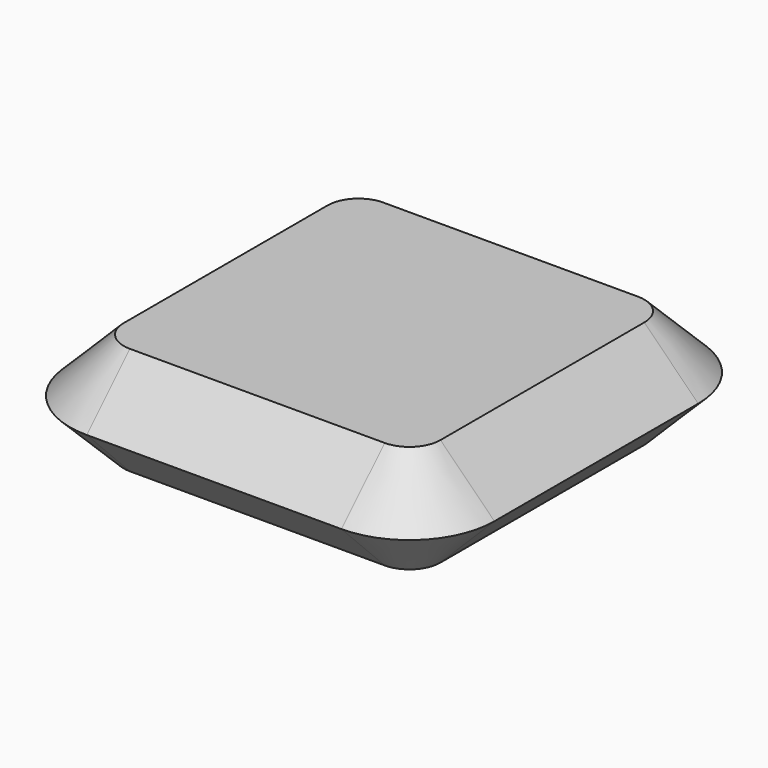
from build123d import *

# Parameters (mm, degrees)
F1_DEPTH = 25.4
F2_SIZE  = 12.7
F3_SIZE  = 12.69999


# Not quite as in the source:
# - a fillet or chamfer is up to 0.001 mm smaller than in the source, because OpenCascade refuses the exact size


with BuildPart() as f1:
    # F0 (on Top) → F1 (new body)
    with BuildSketch(Plane.XY):
        with BuildLine():
            Line((-30, -50), (30, -50))
            ThreePointArc((30, -50), (44.1421356237, -44.1421356237), (50, -30))
            Line((50, -30), (50, 30))
            ThreePointArc((50, 30), (44.1421356237, 44.1421356237), (30, 50))
            Line((30, 50), (-30, 50))
            ThreePointArc((-30, 50), (-44.1421356237, 44.1421356237), (-50, 30))
            Line((-50, 30), (-50, -30))
            ThreePointArc((-50, -30), (-44.1421356237, -44.1421356237), (-30, -50))
        make_face()
    extrude(amount=F1_DEPTH)

    # F2
    f2_edges = [f1.edges().sort_by_distance(p)[0] for p in [
        (0, -50, 25.4),
        (44.142136, -44.142136, 25.4),
        (50, 0, 25.4),
        (44.142136, 44.142136, 25.4),
        (0, 50, 25.4),
        (-44.142136, 44.142136, 25.4),
        (-50, 0, 25.4),
        (-44.142136, -44.142136, 25.4),
    ]]
    chamfer(f2_edges, length=F2_SIZE)

    # F3 (size 12.7 in the source; OpenCascade refuses exactly that, so slightly less here)
    f3_edges = [f1.edges().sort_by_distance(p)[0] for p in [
        (0, -50, 0),
        (44.142136, -44.142136, 0),
        (50, 0, 0),
        (44.142136, 44.142136, 0),
        (0, 50, 0),
        (-44.142136, 44.142136, 0),
        (-50, 0, 0),
        (-44.142136, -44.142136, 0),
    ]]
    chamfer(f3_edges, length=F3_SIZE)


solid = f1.part
